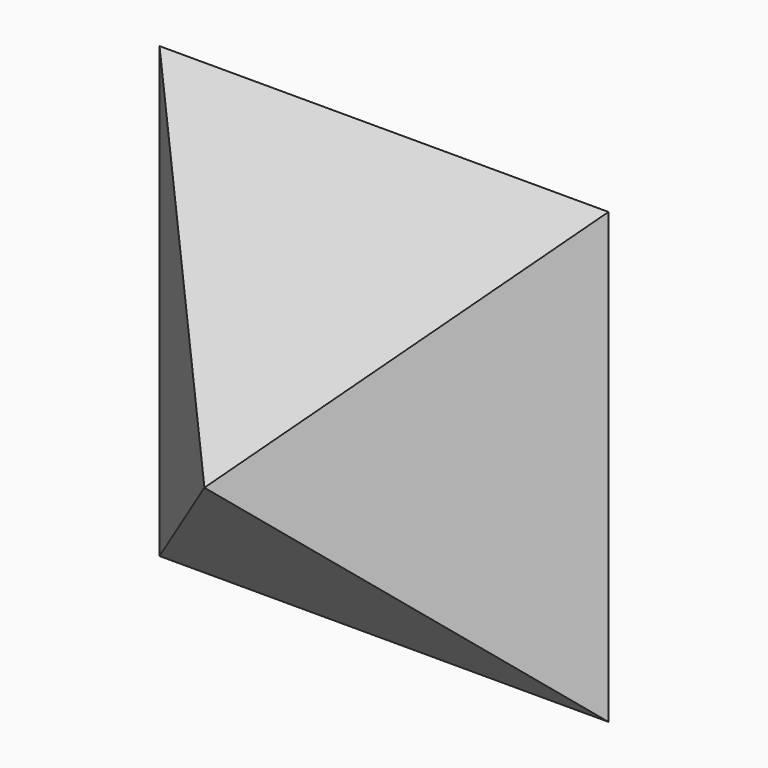
from build123d import *

# Parameters (mm, degrees)
F0_W     = 10
F0_H     = 10
F1_DEPTH = 5
F2_SIZE2 = 4.99999
F2_SIZE  = 4.99999


# Not quite as in the source:
# - a fillet or chamfer is up to 0.001 mm smaller than in the source, because OpenCascade refuses the exact size
# - a feature names something its author has since deleted; it is built from what else it names


with BuildPart() as f1:
    # F0 (on Front) → F1 (new body, symmetric)
    with BuildSketch(Plane.XZ):
        Rectangle(F0_W, F0_H)
    extrude(amount=F1_DEPTH, both=True)

    # F2 (size 5 and 5 in the source; OpenCascade refuses exactly that, so slightly less here)
    f2_edges = [f1.edges().sort_by_distance(p)[0] for p in [
        (0, -5, 5),
        (-5, -5, 0),
        (0, -5, -5),
        (5, -5, 0),
        (0, 5, 5),
        (-5, 5, 0),
        (0, 5, -5),
        (5, 5, 0),
    ]]
    chamfer(f2_edges, length=F2_SIZE, length2=F2_SIZE2)


solid = f1.part
